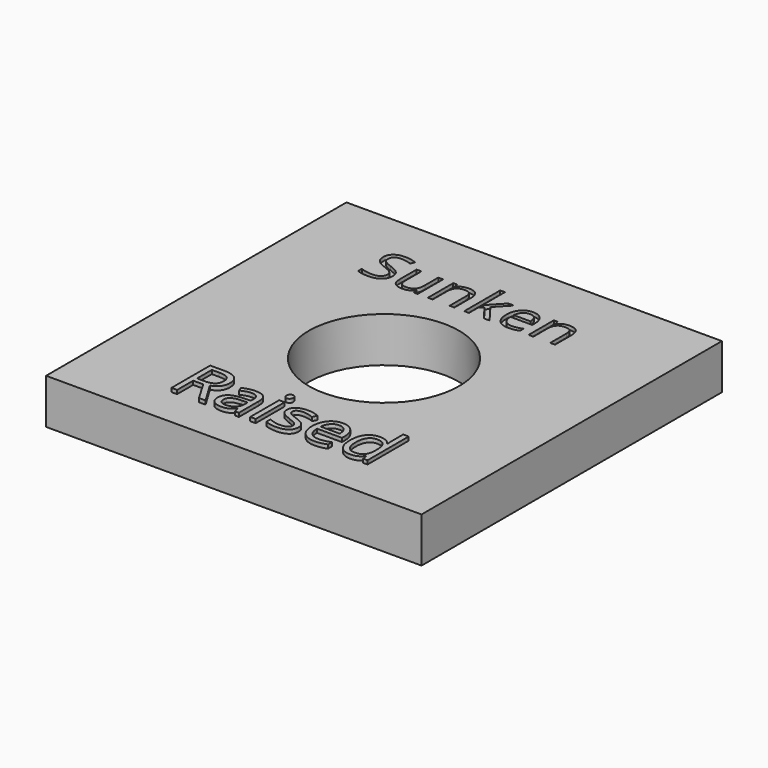
from build123d import *

# Parameters (mm, degrees)
F0_W         = 25
F0_H         = 25
F1_DEPTH     = 3
F2_D         = 10
F3_TEXT_SIZE = 3.94179434
F4_DEPTH     = 0.2525
F5_TEXT_SIZE = 4.5100712062
F6_DEPTH     = 0.25


# Not quite as in the source:
# - Text() gives the source's letters only with a copy of the font that has no kerning and outlines rounded to 1/6400 em; it was checked with that copy


with BuildPart() as f1:
    # F0 (on Top) → F1 (new body)
    with BuildSketch(Plane.XY):
        Rectangle(F0_W, F0_H)
    extrude(amount=F1_DEPTH)

    # F2 (through all)
    with Locations(Plane(origin=(0, 0, 0), x_dir=(1, 0, 0), z_dir=(0, 0, -1))):
        with Locations((0, 0)):
            Hole(F2_D / 2)

    # F3 (on face) → F4 (cut)
    with BuildSketch(Plane.XY.offset(3)):
        with Locations((-7.4071417621, 6.7599234171)):
            Text('Sunken', F3_TEXT_SIZE, font='Open Sans', text_align=(TextAlign.LEFT, TextAlign.BOTTOM))
    extrude(amount=-F4_DEPTH, mode=Mode.SUBTRACT)

    # F5 (on face) → F6 (join)
    with BuildSketch(Plane.XY.offset(3)):
        with Locations((-6.7000264535, -9.8650683649)):
            Text('Raised', F5_TEXT_SIZE, font='Open Sans', text_align=(TextAlign.LEFT, TextAlign.BOTTOM))
    extrude(amount=F6_DEPTH)


solid = f1.part
